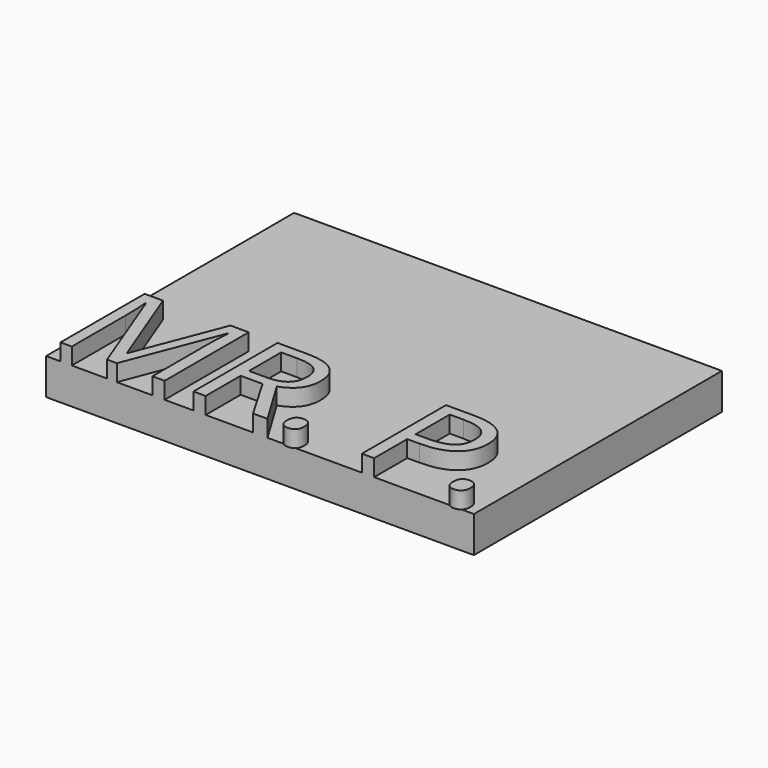
from build123d import *

# Parameters (mm, degrees)
F0_W         = 65
F0_H         = 47.1067047374
F1_DEPTH     = 5.5
F2_TEXT_SIZE = 22.370402237
F3_DEPTH     = 2.54


# Not quite as in the source:
# - Text() gives the source's letters only with a copy of the font that has no kerning and outlines rounded to 1/6400 em; it was checked with that copy


with BuildPart() as f1:
    # F0 (on Top) → F1 (new body)
    with BuildSketch(Plane.XY):
        Rectangle(F0_W, F0_H)
    extrude(amount=F1_DEPTH)

    # F2 (on face) → F3 (join)
    with BuildSketch(Plane.XY.offset(5.5)):
        with Locations((-32.5, -23.5533523687)):
            Text('MR. P.', F2_TEXT_SIZE, font='Open Sans', text_align=(TextAlign.LEFT, TextAlign.BOTTOM))
    extrude(amount=F3_DEPTH)


solid = f1.part
